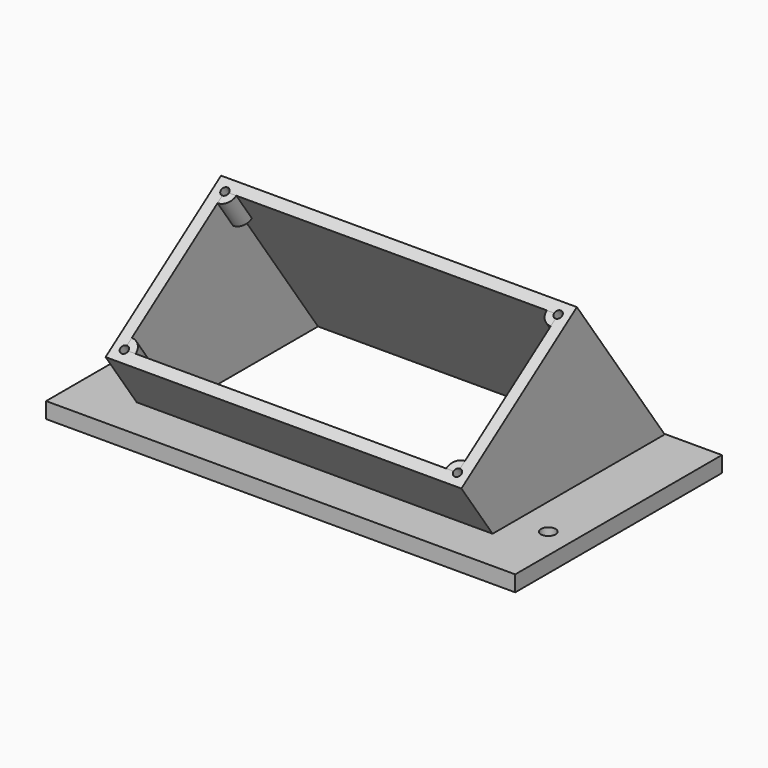
from build123d import *

# Parameters (mm, degrees)
F0_R          = 3.25
F0_W          = 147
F0_H          = 74
F0_W_2        = 5
F0_H_2        = 3
F1_DEPTH      = 7
F4_DEPTH      = 150.739
F4_DEPTH_BACK = 6.261
F5_W          = 147
F5_H          = 67.7437671193
F6_DEPTH      = 156.2
F7_R          = 1
F9_DEPTH      = 15
F10_R         = 1.75
F11_DEPTH     = 15


# Not quite as in the source:
# - a feature names something its author has since deleted; it is built from what else it names


with BuildPart() as f1:
    # F0 (on Top) → F1 (new body)
    with BuildSketch(Plane.XY):
        Polygon((30.7393903136, 82), (-31.2606096864, 82), (-31.2606096864, -32), (175.7393903136, -32), (175.7393903136, 82), (113.7393903136, 82), (108.7393903136, 82), (35.7393903136, 82), align=None)
        with Locations((-20.2606096864, 0)):
            Circle(F0_R, mode=Mode.SUBTRACT)
        with Locations((164.7393903136, 0)):
            Circle(F0_R, mode=Mode.SUBTRACT)
        with Locations((72.2393903136, 30)):
            Rectangle(F0_W, F0_H, mode=Mode.SUBTRACT)
        with Locations((33.2393903136, 83.5)):
            Rectangle(F0_W_2, F0_H_2)
        with Locations((111.2393903136, 83.5)):
            Rectangle(F0_W_2, F0_H_2)
    extrude(amount=F1_DEPTH)

    # F3 (on Right) → F4 (join, two sides)
    with BuildSketch(Plane.YZ) as f4_sk:
        Polygon((-13.2231451571, 7), (81.6844701767, 7), (33.2535275188, 76.1665542214), (-30.4304382476, 31.5745613287), align=None)
    extrude(amount=F4_DEPTH)
    extrude(f4_sk.sketch, amount=-F4_DEPTH_BACK)

    # F5 (on face) → F6 (cut)
    with BuildSketch(Plane(origin=(0, -24.8464988409, 35.4844777942), x_dir=(1, 0, 0), z_dir=(0, -0.5735764364, 0.8191520443))):
        with Locations((72.239, 32.0551522267)):
            Rectangle(F5_W, F5_H)
    extrude(amount=-F6_DEPTH, mode=Mode.SUBTRACT)

    # F7
    f7_edges = [f1.edges().sort_by_distance(p)[0] for p in [
        (111.23939, 85, 7),
        (33.23939, 85, 7),
        (35.73939, 85, 3.5),
        (30.73939, 85, 3.5),
        (108.73939, 85, 3.5),
        (113.73939, 85, 3.5),
    ]]
    fillet(f7_edges, radius=F7_R)

    # F8 (on face) → F9 (join)
    with BuildSketch(Plane(origin=(0, -24.8464988409, 35.4844777942), x_dir=(1, 0, 0), z_dir=(0, -0.5735764364, 0.8191520443))):
        with BuildLine():
            Line((-1.261, 65.9270357864), (3.739, 65.9270357864))
            ThreePointArc((3.739, 65.9270357864), (2.2745339059, 69.4625696923), (-1.261, 70.9270357864))
            Line((-1.261, 70.9270357864), (-6.261, 70.9270357864))
            Line((-6.261, 70.9270357864), (-6.261, 65.9270357864))
            ThreePointArc((-6.261, 65.9270357864), (-4.7965339059, 62.3915018804), (-1.261, 60.9270357864))
            Line((-1.261, 60.9270357864), (-1.261, 65.9270357864))
        make_face()
        with BuildLine():
            ThreePointArc((-1.261, 60.9270357864), (2.2745339059, 62.3915018804), (3.739, 65.9270357864))
            Line((3.739, 65.9270357864), (-1.261, 65.9270357864))
            Line((-1.261, 65.9270357864), (-1.261, 60.9270357864))
        make_face()
        with BuildLine():
            Line((145.739, -1.8167313329), (145.739, 3.1832686671))
            ThreePointArc((145.739, 3.1832686671), (142.2034660941, 1.718802573), (140.739, -1.8167313329))
            Line((140.739, -1.8167313329), (145.739, -1.8167313329))
        make_face()
        with BuildLine():
            ThreePointArc((140.739, 65.9270357864), (142.2034660941, 62.3915018804), (145.739, 60.9270357864))
            Line((145.739, 60.9270357864), (145.739, 65.9270357864))
            Line((145.739, 65.9270357864), (140.739, 65.9270357864))
        make_face()
        with BuildLine():
            Line((150.739, -6.8167313329), (150.739, -1.8167313329))
            ThreePointArc((150.739, -1.8167313329), (149.2745339059, 1.718802573), (145.739, 3.1832686671))
            Line((145.739, 3.1832686671), (145.739, -1.8167313329))
            Line((145.739, -1.8167313329), (140.739, -1.8167313329))
            ThreePointArc((140.739, -1.8167313329), (142.2034660941, -5.3522652388), (145.739, -6.8167313329))
            Line((145.739, -6.8167313329), (150.739, -6.8167313329))
        make_face()
        with BuildLine():
            ThreePointArc((145.739, 60.9270357864), (149.2745339059, 62.3915018804), (150.739, 65.9270357864))
            Line((150.739, 65.9270357864), (150.739, 70.9270357864))
            Line((150.739, 70.9270357864), (145.739, 70.9270357864))
            ThreePointArc((145.739, 70.9270357864), (142.2034660941, 69.4625696923), (140.739, 65.9270357864))
            Line((140.739, 65.9270357864), (145.739, 65.9270357864))
            Line((145.739, 65.9270357864), (145.739, 60.9270357864))
        make_face()
        with BuildLine():
            Line((-1.261, -1.8167313329), (3.739, -1.8167313329))
            ThreePointArc((3.739, -1.8167313329), (2.2745339059, 1.718802573), (-1.261, 3.1832686671))
            Line((-1.261, 3.1832686671), (-1.261, -1.8167313329))
        make_face()
    extrude(amount=-F9_DEPTH)

    # F10 (on face) → F11 (cut)
    with BuildSketch(Plane(origin=(0, -24.8464988409, 35.4844777942), x_dir=(1, 0, 0), z_dir=(0, -0.5735764364, 0.8191520443))):
        with Locations((145.739, -1.8167313329)):
            Circle(F10_R)
        with Locations((145.739, 65.9270357864)):
            Circle(F10_R)
        with Locations((-1.261, 65.9270357864)):
            Circle(F10_R)
        with Locations((-1.261, -1.8167313329)):
            Circle(F10_R)
    extrude(amount=-F11_DEPTH, mode=Mode.SUBTRACT)


solid = f1.part
